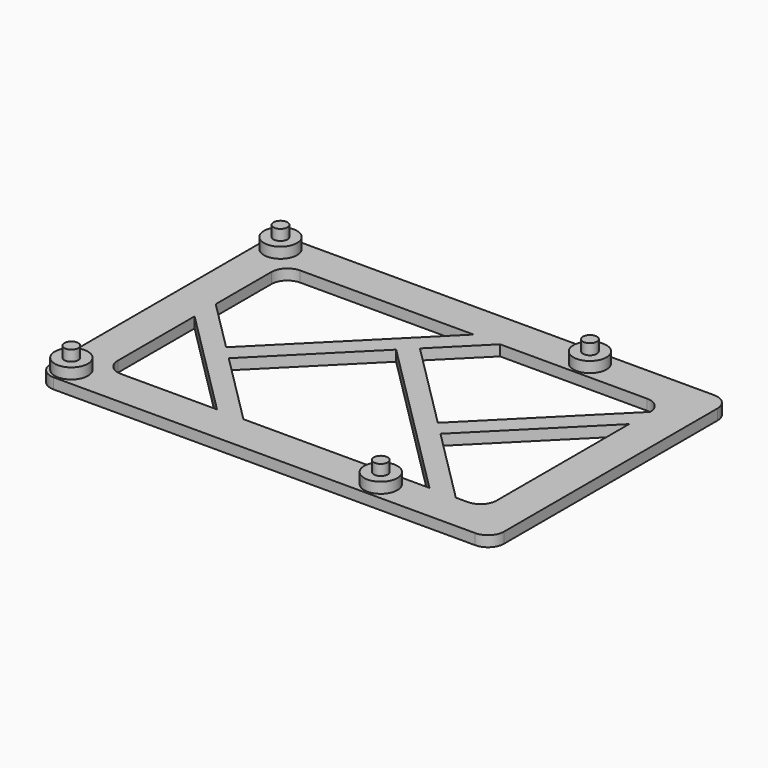
from build123d import *

# Parameters (mm, degrees)
F0_R     = 3.1
F0_R_2   = 1.3
F1_DEPTH = 4
F2_DEPTH = 2
F3_DEPTH = 6


with BuildPart() as f1:
    # F0 (on Top) → F1 (new body)
    with BuildSketch(Plane.XY):
        with Locations((-39, -24.5)):
            Circle(F0_R)
        with Locations((-39, -24.5)):
            Circle(F0_R_2, mode=Mode.SUBTRACT)
    extrude(amount=F1_DEPTH)


with BuildPart() as f1b:
    # F0 (on Top) → F1, piece 2 (new body)
    with BuildSketch(Plane.XY):
        with Locations((19, -24.5)):
            Circle(F0_R)
        with Locations((19, -24.5)):
            Circle(F0_R_2, mode=Mode.SUBTRACT)
    extrude(amount=F1_DEPTH)

    # F0 (on Top) → F3 (join)
    with BuildSketch(Plane.XY):
        with Locations((19, -24.5)):
            Circle(F0_R_2)
    extrude(amount=F3_DEPTH)


with BuildPart() as f1c:
    # F0 (on Top) → F1, piece 3 (new body)
    with BuildSketch(Plane.XY):
        with Locations((-39, 24.5)):
            Circle(F0_R)
        with Locations((-39, 24.5)):
            Circle(F0_R_2, mode=Mode.SUBTRACT)
    extrude(amount=F1_DEPTH)


with BuildPart() as f1d:
    # F0 (on Top) → F1, piece 4 (new body)
    with BuildSketch(Plane.XY):
        with Locations((19, 24.5)):
            Circle(F0_R)
        with Locations((19, 24.5)):
            Circle(F0_R_2, mode=Mode.SUBTRACT)
    extrude(amount=F1_DEPTH)


with BuildPart() as f2:
    # F0 (on Top) → F2 (new body)
    with BuildSketch(Plane.XY):
        with BuildLine():
            Line((39.5, 28), (-39.5, 28))
            ThreePointArc((-39.5, 28), (-41.6213203436, 27.1213203436), (-42.5, 25))
            Line((-42.5, 25), (-42.5, -25))
            ThreePointArc((-42.5, -25), (-41.6213203436, -27.1213203436), (-39.5, -28))
            Line((-39.5, -28), (39.5, -28))
            ThreePointArc((39.5, -28), (41.6213203436, -27.1213203436), (42.5, -25))
            Line((42.5, -25), (42.5, 25))
            ThreePointArc((42.5, 25), (41.6213203436, 27.1213203436), (39.5, 28))
        make_face()
        with Locations((-39, -24.5)):
            Circle(F0_R, mode=Mode.SUBTRACT)
        with Locations((19, -24.5)):
            Circle(F0_R, mode=Mode.SUBTRACT)
        with Locations((-39, 24.5)):
            Circle(F0_R, mode=Mode.SUBTRACT)
        with BuildLine():
            ThreePointArc((-35.5, 18), (-34.6213203436, 20.1213203436), (-32.5, 21))
            Line((-32.5, 21), (0, 21))
            Line((0, 21), (4.9497474683, 21))
            Line((4.9497474683, 21), (32.5, 21))
            ThreePointArc((32.5, 21), (34.6213203436, 20.1213203436), (35.5, 18))
            Line((35.5, 18), (35.5, 13.0502525317))
            Line((35.5, 13.0502525317), (35.5, -18))
            ThreePointArc((35.5, -18), (34.6213203436, -20.1213203436), (32.5, -21))
            Line((32.5, -21), (30.2628741404, -21))
            Line((30.2628741404, -21), (25.3131266721, -21))
            Line((25.3131266721, -21), (-9.5502525317, -21))
            Line((-9.5502525317, -21), (-14.5, -21))
            Line((-14.5, -21), (-32.5, -21))
            ThreePointArc((-32.5, -21), (-34.6213203436, -20.1213203436), (-35.5, -18))
            Line((-35.5, -18), (-35.5, 0))
            Line((-35.5, 0), (-35.5, 4.9497474683))
            Line((-35.5, 4.9497474683), (-35.5, 18))
        make_face(mode=Mode.SUBTRACT)
        with Locations((19, 24.5)):
            Circle(F0_R, mode=Mode.SUBTRACT)
        Polygon((4.9497474683, 21), (0, 21), (-25.7751262658, -4.7751262658), (-23.3002525317, -7.25), (-5.8685629298, 10.1816896019), (-3.3936891957, 12.656563336), align=None)
        Polygon((-23.3002525317, -7.25), (-25.7751262658, -4.7751262658), (-35.5, 4.9497474683), (-35.5, 0), (-14.5, -21), (-9.5502525317, -21), align=None)
        Polygon((13.3814370702, -4.1185629298), (-3.3936891957, 12.656563336), (-5.8685629298, 10.1816896019), (25.3131266721, -21), (30.2628741404, -21), (15.8563108043, -6.593436664), align=None)
        Polygon((35.5, 13.0502525317), (35.5, 18), (13.3814370702, -4.1185629298), (15.8563108043, -6.593436664), align=None)
    extrude(amount=F2_DEPTH)


with BuildPart() as f3:
    # F0 (on Top) → F3, piece 2 (new body)
    with BuildSketch(Plane.XY):
        with Locations((-39, -24.5)):
            Circle(F0_R_2)
    extrude(amount=F3_DEPTH)


with BuildPart() as f3b:
    # F0 (on Top) → F3, piece 3 (new body)
    with BuildSketch(Plane.XY):
        with Locations((-39, 24.5)):
            Circle(F0_R_2)
    extrude(amount=F3_DEPTH)


with BuildPart() as f3c:
    # F0 (on Top) → F3, piece 4 (new body)
    with BuildSketch(Plane.XY):
        with Locations((19, 24.5)):
            Circle(F0_R_2)
    extrude(amount=F3_DEPTH)


solid = Compound([f1.part, f1b.part, f1c.part, f1d.part, f2.part, f3.part, f3b.part, f3c.part])
